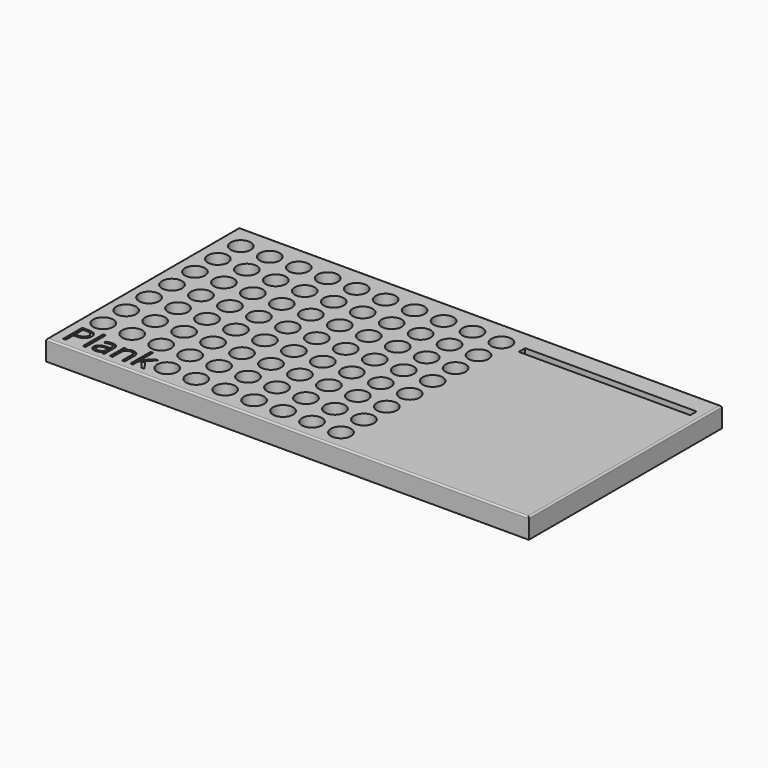
from build123d import *

# Parameters (mm, degrees)
F0_W         = 600
F0_H         = 300
F0_R         = 12.5
F0_W_2       = 213.1477892399
F0_H_2       = 10
F1_DEPTH     = 25
F2_DEPTH     = 15
F3_R         = 2
F4_TEXT_SIZE = 41.4555167986
F5_DEPTH     = 2


# Not quite as in the source:
# - Text() gives the source's letters only with a copy of the font that has no kerning and outlines rounded to 1/6400 em; it was checked with that copy


with BuildPart() as f1:
    # F0 (on Top) → F1 (new body)
    with BuildSketch(Plane.XY):
        Rectangle(F0_W, F0_H)
        with Locations((-169.5, -124.9749987244)):
            Circle(F0_R, mode=Mode.SUBTRACT)
        with Locations((-277, -89.9785703352)):
            Circle(F0_R, mode=Mode.SUBTRACT)
        with Locations((-241, -89.9785703352)):
            Circle(F0_R, mode=Mode.SUBTRACT)
        with Locations((-205, -89.9785703352)):
            Circle(F0_R, mode=Mode.SUBTRACT)
        with Locations((-169, -89.9785703352)):
            Circle(F0_R, mode=Mode.SUBTRACT)
        with Locations((-133.5, -124.9749987244)):
            Circle(F0_R, mode=Mode.SUBTRACT)
        with Locations((-97.5, -124.9749987244)):
            Circle(F0_R, mode=Mode.SUBTRACT)
        with Locations((-61.5, -124.9749987244)):
            Circle(F0_R, mode=Mode.SUBTRACT)
        with Locations((-25.5, -124.9749987244)):
            Circle(F0_R, mode=Mode.SUBTRACT)
        with Locations((-133, -89.9785703352)):
            Circle(F0_R, mode=Mode.SUBTRACT)
        with Locations((-97, -89.9785703352)):
            Circle(F0_R, mode=Mode.SUBTRACT)
        with Locations((-61, -89.9785703352)):
            Circle(F0_R, mode=Mode.SUBTRACT)
        with Locations((-25, -89.9785703352)):
            Circle(F0_R, mode=Mode.SUBTRACT)
        with Locations((-276.5, -54.982141946)):
            Circle(F0_R, mode=Mode.SUBTRACT)
        with Locations((-240.5, -54.982141946)):
            Circle(F0_R, mode=Mode.SUBTRACT)
        with Locations((-204.5, -54.982141946)):
            Circle(F0_R, mode=Mode.SUBTRACT)
        with Locations((-168.5, -54.982141946)):
            Circle(F0_R, mode=Mode.SUBTRACT)
        with Locations((-276, -19.9857135568)):
            Circle(F0_R, mode=Mode.SUBTRACT)
        with Locations((-240, -19.9857135568)):
            Circle(F0_R, mode=Mode.SUBTRACT)
        with Locations((-204, -19.9857135568)):
            Circle(F0_R, mode=Mode.SUBTRACT)
        with Locations((-168, -19.9857135568)):
            Circle(F0_R, mode=Mode.SUBTRACT)
        with Locations((-132.5, -54.982141946)):
            Circle(F0_R, mode=Mode.SUBTRACT)
        with Locations((-96.5, -54.982141946)):
            Circle(F0_R, mode=Mode.SUBTRACT)
        with Locations((-60.5, -54.982141946)):
            Circle(F0_R, mode=Mode.SUBTRACT)
        with Locations((-24.5, -54.982141946)):
            Circle(F0_R, mode=Mode.SUBTRACT)
        with Locations((-132, -19.9857135568)):
            Circle(F0_R, mode=Mode.SUBTRACT)
        with Locations((-96, -19.9857135568)):
            Circle(F0_R, mode=Mode.SUBTRACT)
        with Locations((-60, -19.9857135568)):
            Circle(F0_R, mode=Mode.SUBTRACT)
        with Locations((-24, -19.9857135568)):
            Circle(F0_R, mode=Mode.SUBTRACT)
        with Locations((10.5, -124.9749987244)):
            Circle(F0_R, mode=Mode.SUBTRACT)
        with Locations((46.5, -124.9749987244)):
            Circle(F0_R, mode=Mode.SUBTRACT)
        with Locations((11, -89.9785703352)):
            Circle(F0_R, mode=Mode.SUBTRACT)
        with Locations((47, -89.9785703352)):
            Circle(F0_R, mode=Mode.SUBTRACT)
        with Locations((11.5, -54.982141946)):
            Circle(F0_R, mode=Mode.SUBTRACT)
        with Locations((47.5, -54.982141946)):
            Circle(F0_R, mode=Mode.SUBTRACT)
        with Locations((12, -19.9857135568)):
            Circle(F0_R, mode=Mode.SUBTRACT)
        with Locations((48, -19.9857135568)):
            Circle(F0_R, mode=Mode.SUBTRACT)
        with Locations((-275.5, 15.0107148324)):
            Circle(F0_R, mode=Mode.SUBTRACT)
        with Locations((-239.5, 15.0107148324)):
            Circle(F0_R, mode=Mode.SUBTRACT)
        with Locations((-203.5, 15.0107148324)):
            Circle(F0_R, mode=Mode.SUBTRACT)
        with Locations((-167.5, 15.0107148324)):
            Circle(F0_R, mode=Mode.SUBTRACT)
        with Locations((-275, 50.0071432216)):
            Circle(F0_R, mode=Mode.SUBTRACT)
        with Locations((-239, 50.0071432216)):
            Circle(F0_R, mode=Mode.SUBTRACT)
        with Locations((-203, 50.0071432216)):
            Circle(F0_R, mode=Mode.SUBTRACT)
        with Locations((-167, 50.0071432216)):
            Circle(F0_R, mode=Mode.SUBTRACT)
        with Locations((-131.5, 15.0107148324)):
            Circle(F0_R, mode=Mode.SUBTRACT)
        with Locations((-95.5, 15.0107148324)):
            Circle(F0_R, mode=Mode.SUBTRACT)
        with Locations((-59.5, 15.0107148324)):
            Circle(F0_R, mode=Mode.SUBTRACT)
        with Locations((-23.5, 15.0107148324)):
            Circle(F0_R, mode=Mode.SUBTRACT)
        with Locations((-131, 50.0071432216)):
            Circle(F0_R, mode=Mode.SUBTRACT)
        with Locations((-95, 50.0071432216)):
            Circle(F0_R, mode=Mode.SUBTRACT)
        with Locations((-59, 50.0071432216)):
            Circle(F0_R, mode=Mode.SUBTRACT)
        with Locations((-23, 50.0071432216)):
            Circle(F0_R, mode=Mode.SUBTRACT)
        with Locations((-274.5, 85.0035716108)):
            Circle(F0_R, mode=Mode.SUBTRACT)
        with Locations((-238.5, 85.0035716108)):
            Circle(F0_R, mode=Mode.SUBTRACT)
        with Locations((-202.5, 85.0035716108)):
            Circle(F0_R, mode=Mode.SUBTRACT)
        with Locations((-166.5, 85.0035716108)):
            Circle(F0_R, mode=Mode.SUBTRACT)
        with Locations((-274, 120)):
            Circle(F0_R, mode=Mode.SUBTRACT)
        with Locations((-238, 120)):
            Circle(F0_R, mode=Mode.SUBTRACT)
        with Locations((-202, 120)):
            Circle(F0_R, mode=Mode.SUBTRACT)
        with Locations((-166, 120)):
            Circle(F0_R, mode=Mode.SUBTRACT)
        with Locations((-130.5, 85.0035716108)):
            Circle(F0_R, mode=Mode.SUBTRACT)
        with Locations((-94.5, 85.0035716108)):
            Circle(F0_R, mode=Mode.SUBTRACT)
        with Locations((-58.5, 85.0035716108)):
            Circle(F0_R, mode=Mode.SUBTRACT)
        with Locations((-22.5, 85.0035716108)):
            Circle(F0_R, mode=Mode.SUBTRACT)
        with Locations((-130, 120)):
            Circle(F0_R, mode=Mode.SUBTRACT)
        with Locations((-94, 120)):
            Circle(F0_R, mode=Mode.SUBTRACT)
        with Locations((-58, 120)):
            Circle(F0_R, mode=Mode.SUBTRACT)
        with Locations((-22, 120)):
            Circle(F0_R, mode=Mode.SUBTRACT)
        with Locations((12.5, 15.0107148324)):
            Circle(F0_R, mode=Mode.SUBTRACT)
        with Locations((48.5, 15.0107148324)):
            Circle(F0_R, mode=Mode.SUBTRACT)
        with Locations((13, 50.0071432216)):
            Circle(F0_R, mode=Mode.SUBTRACT)
        with Locations((49, 50.0071432216)):
            Circle(F0_R, mode=Mode.SUBTRACT)
        with Locations((13.5, 85.0035716108)):
            Circle(F0_R, mode=Mode.SUBTRACT)
        with Locations((49.5, 85.0035716108)):
            Circle(F0_R, mode=Mode.SUBTRACT)
        with Locations((14, 120)):
            Circle(F0_R, mode=Mode.SUBTRACT)
        with Locations((50, 120)):
            Circle(F0_R, mode=Mode.SUBTRACT)
        with Locations((182, 120)):
            Rectangle(F0_W_2, F0_H_2, mode=Mode.SUBTRACT)
    extrude(amount=F1_DEPTH)

    # F0 (on Top) → F2 (join)
    with BuildSketch(Plane.XY):
        with Locations((182, 120)):
            Rectangle(F0_W_2, F0_H_2)
    extrude(amount=F2_DEPTH)

    # F3
    f3_edges = [f1.edges().sort_by_distance(p)[0] for p in [
        (0, 150, 25),
        (-300, 0, 25),
        (0, -150, 25),
        (300, 0, 25),
    ]]
    fillet(f3_edges, radius=F3_R)

    # F4 (on face) → F5 (cut)
    with BuildSketch(Plane.XY.offset(25)):
        with Locations((-291.0465598106, -139.7597491741)):
            Text('Plank', F4_TEXT_SIZE, font='Open Sans', text_align=(TextAlign.LEFT, TextAlign.BOTTOM))
    extrude(amount=-F5_DEPTH, mode=Mode.SUBTRACT)


solid = f1.part
